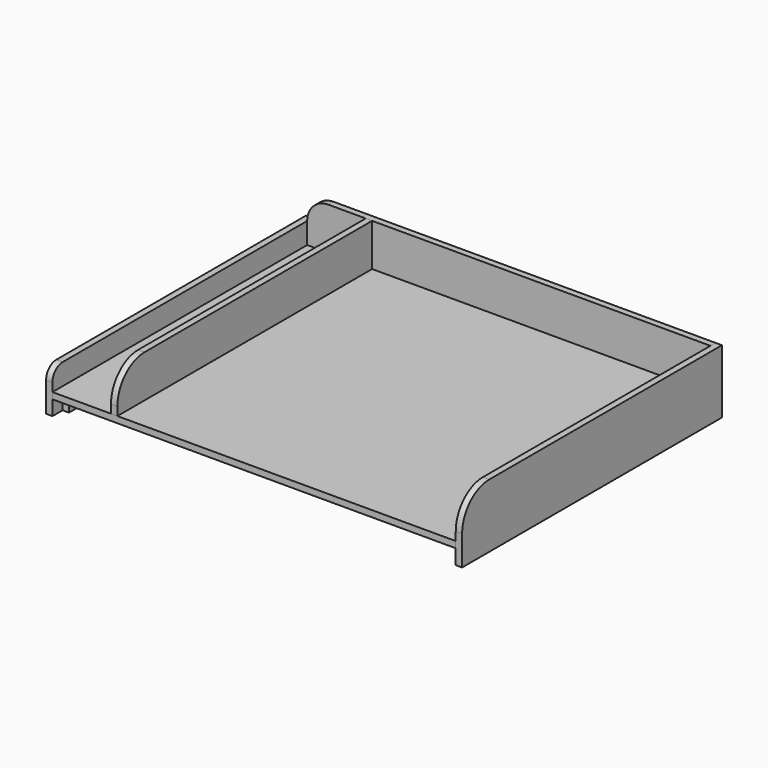
from build123d import *

# Parameters (mm, degrees)
F0_W      = 950
F0_H      = 750
F1_DEPTH  = 15
F2_W      = 750
F2_H      = 15
F3_DEPTH  = 15
F4_R      = 80
F5_W      = 765
F5_H      = 100
F6_DEPTH  = 15
F7_R      = 30
F8_W      = 15
F8_H      = 750
F9_DEPTH  = 100
F10_R     = 80
F11_W     = 950
F11_H     = 150
F12_DEPTH = 15
F13_R     = 50
F14_W     = 15
F14_H     = 15
F15_DEPTH = 720


# Not quite as in the source:
# - a feature names something its author has since deleted; it is built from what else it names


with BuildPart() as f1:
    # F0 (on Top) → F1 (new body)
    with BuildSketch(Plane.XY):
        with Locations((475, 375)):
            Rectangle(F0_W, F0_H)
    extrude(amount=F1_DEPTH)


with BuildPart() as f3:
    # F2 (on face) → F3 (new body)
    with BuildSketch(Plane.YZ.offset(950)):
        Polygon((0, 0), (0, -35), (765, -35), (765, 115), (0, 115), (0, 15), (750, 15), (750, 0), align=None)
        with Locations((375, 7.5)):
            Rectangle(F2_W, F2_H)
    extrude(amount=F3_DEPTH)

    # F4
    f4_edges = [f3.edges().sort_by_distance(p)[0] for p in [
        (957.5, 0, 115),
    ]]
    fillet(f4_edges, radius=F4_R)


with BuildPart() as f6:
    # F5 (on face) → F6 (new body)
    with BuildSketch(Plane(origin=(0, 0, 0), x_dir=(0, -1, 0), z_dir=(-1, 0, 0))):
        with Locations((-382.5, 15)):
            Rectangle(F5_W, F5_H)
    extrude(amount=F6_DEPTH)

    # F7
    f7_edges = [f6.edges().sort_by_distance(p)[0] for p in [
        (-7.5, 0, 65),
    ]]
    fillet(f7_edges, radius=F7_R)


with BuildPart() as f9:
    # F8 (on face) → F9 (new body)
    with BuildSketch(Plane.XY.offset(15)):
        with Locations((145.5, 375)):
            Rectangle(F8_W, F8_H)
    extrude(amount=F9_DEPTH)

    # F10
    f10_edges = [f9.edges().sort_by_distance(p)[0] for p in [
        (145.5, 0, 115),
    ]]
    fillet(f10_edges, radius=F10_R)


with BuildPart() as f12:
    # F11 (on face) → F12 (new body)
    with BuildSketch(Plane(origin=(0, 750, 0), x_dir=(-1, 0, 0), z_dir=(0, 1, 0))):
        with Locations((-475, 40)):
            Rectangle(F11_W, F11_H)
    extrude(amount=F12_DEPTH)

    # F13
    f13_edges = [f12.edges().sort_by_distance(p)[0] for p in [
        (0, 757.5, 115),
    ]]
    fillet(f13_edges, radius=F13_R)


with BuildPart() as f15:
    # F14 (on face) → F15 (new body)
    with BuildSketch(Plane.XZ.offset(-750)):
        with Locations((7.5, -27.5)):
            Rectangle(F14_W, F14_H)
    extrude(amount=F15_DEPTH)


with BuildPart() as f15b:
    # F14 (on face) → F15, piece 2 (new body)
    with BuildSketch(Plane.XZ.offset(-750)):
        with Locations((942.5, -27.5)):
            Rectangle(F14_W, F14_H)
    extrude(amount=F15_DEPTH)


solid = Compound([f1.part, f3.part, f6.part, f9.part, f12.part, f15.part, f15b.part])
